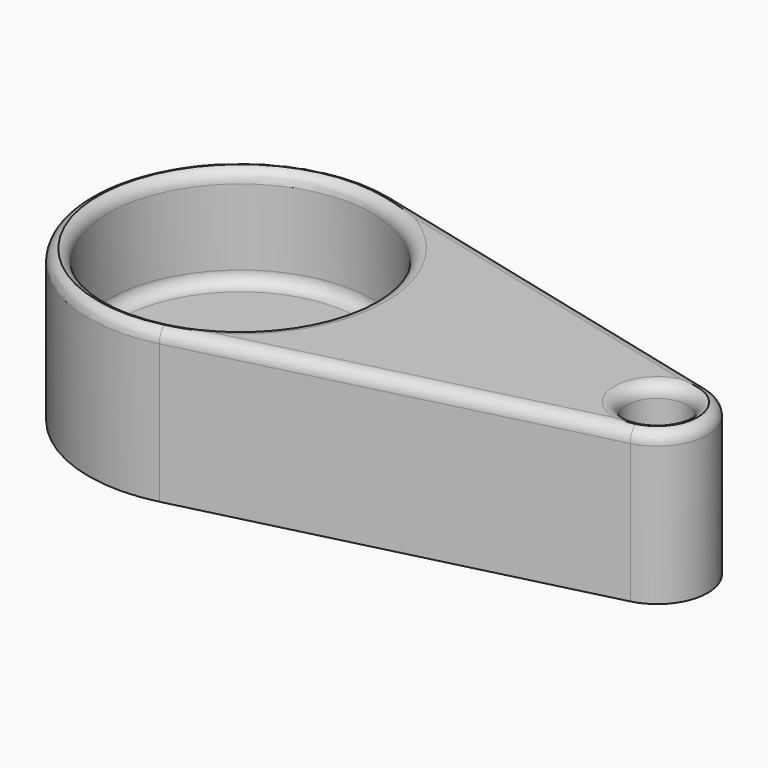
from build123d import *

# Parameters (mm, degrees)
F1_DEPTH     = 30
F2_R         = 26.25
F2_R_2       = 6
F3_DEPTH     = 20
F4_T5_DEPTH  = 80
F4_T7_DEPTH  = 80
F4_T10_ANGLE = 208.0724869359
F4_T12_ANGLE = 151.9275130641
F5_T         = -1


# Not quite as in the source:
# - a fillet or chamfer that OpenCascade refuses, or shapes differently, is made with other operations: its cross-section is extruded or revolved along the edge and cut away or added


with BuildPart() as f1:
    # F0 (on Top) → F1 (new body)
    with BuildSketch(Plane.XY):
        with BuildLine():
            ThreePointArc((-78.9887374496, -29.1042750044), (-62.6186430602, -18.4623662821), (-56.2648062007, 0))
            ThreePointArc((-56.2648062007, 0), (-62.6186430602, 18.4623662821), (-78.9887374496, 29.1042750044))
            ThreePointArc((-78.9887374496, 29.1042750044), (-116.2648062007, 0), (-78.9887374496, -29.1042750044))
        make_face()
        with BuildLine():
            ThreePointArc((-78.9887374496, 29.1042750044), (-62.6186430602, 18.4623662821), (-56.2648062007, 0))
            ThreePointArc((-56.2648062007, 0), (-62.6186430602, -18.4623662821), (-78.9887374496, -29.1042750044))
            Line((-78.9887374496, -29.1042750044), (-1.377337438, -9.7014250015))
            ThreePointArc((-1.377337438, -9.7014250015), (-13.8026936884, 0), (-1.377337438, 9.7014250015))
            Line((-1.377337438, 9.7014250015), (-78.9887374496, 29.1042750044))
        make_face()
        with BuildLine():
            ThreePointArc((6.1973063116, 0), (4.0793606918, 6.154122094), (-1.377337438, 9.7014250015))
            ThreePointArc((-1.377337438, 9.7014250015), (-13.8026936884, 0), (-1.377337438, -9.7014250015))
            ThreePointArc((-1.377337438, -9.7014250015), (4.0793606918, -6.154122094), (6.1973063116, 0))
        make_face()
    extrude(amount=F1_DEPTH)

    # F2 (on face) → F3 (cut)
    with BuildSketch(Plane.XY.offset(30)):
        with Locations((-86.2648062007, 0)):
            Circle(F2_R)
        with Locations((-3.8026936884, 0)):
            Circle(F2_R_2)
    extrude(amount=-F3_DEPTH, mode=Mode.SUBTRACT)

    # F4: fillet of radius 2.5 on 8 edges, made by hand

    # F4_s1 → F4_t2 (revolve)
    with BuildSketch(Plane.XZ):
        with BuildLine():
            ThreePointArc((-60.0148062007, 12.5), (-60.7470392478, 10.732233047), (-62.5148062007, 10))
            Line((-62.5148062007, 10), (-60.0148062007, 10))
            Line((-60.0148062007, 10), (-60.0148062007, 12.5))
        make_face()
    revolve(axis=Axis((-86.2648062007, 0, 10), (0, 0, 1)))

    # F4_s3 → F4_t4 (revolve)
    with BuildSketch(Plane.XZ):
        with BuildLine():
            ThreePointArc((2.1973063116, 12.5), (1.4650732646, 10.732233047), (-0.3026936884, 10))
            Line((-0.3026936884, 10), (2.1973063116, 10))
            Line((2.1973063116, 10), (2.1973063116, 12.5))
        make_face()
    revolve(axis=Axis((-3.8026936884, 0, 10), (0, 0, 1)))

    # F4_s6 → F4_t5 (cut)
    with BuildSketch(Plane(origin=(-3.5790058244, 0.8947514561, 0), x_dir=(0, 0, 1), z_dir=(-0.9701425001, 0.242535625, 0))):
        with BuildLine():
            ThreePointArc((27.5, 9.0777113095), (29.267766953, 8.3454782624), (30, 6.5777113095))
            Line((30, 6.5777113095), (30, 9.0777113095))
            Line((30, 9.0777113095), (27.5, 9.0777113095))
        make_face()
    extrude(amount=F4_T5_DEPTH, mode=Mode.SUBTRACT)

    # F4_s8 → F4_t7 (cut)
    with BuildSketch(Plane(origin=(-81.190405836, -20.297601459, 0), x_dir=(0, 0, 1), z_dir=(0.9701425001, 0.242535625, 0))):
        with BuildLine():
            ThreePointArc((27.5, 9.0777113095), (29.267766953, 8.3454782624), (30, 6.5777113095))
            Line((30, 6.5777113095), (30, 9.0777113095))
            Line((30, 9.0777113095), (27.5, 9.0777113095))
        make_face()
    extrude(amount=F4_T7_DEPTH, mode=Mode.SUBTRACT)

    # F4_s9 → F4_t10 (revolve, cut)
    with BuildSketch(Plane(origin=(-81.190405836, 20.297601459, 0), x_dir=(0, 0, 1), z_dir=(0.9701425001, -0.242535625, 0))):
        with BuildLine():
            ThreePointArc((27.5, -9.0777113095), (29.267766953, -8.3454782624), (30, -6.5777113095))
            Line((30, -6.5777113095), (30, -9.0777113095))
            Line((30, -9.0777113095), (27.5, -9.0777113095))
        make_face()
    revolve(axis=Axis((-86.2648062007, 0, 30), (0, 0, 1)), revolution_arc=F4_T10_ANGLE, mode=Mode.SUBTRACT)

    # F4_s11 → F4_t12 (revolve, cut)
    with BuildSketch(Plane(origin=(-3.5790058244, -0.8947514561, 0), x_dir=(0, 0, 1), z_dir=(-0.9701425001, -0.242535625, 0))):
        with BuildLine():
            ThreePointArc((30, -6.5777113095), (29.267766953, -8.3454782624), (27.5, -9.0777113095))
            Line((27.5, -9.0777113095), (30, -9.0777113095))
            Line((30, -9.0777113095), (30, -6.5777113095))
        make_face()
    revolve(axis=Axis((-3.8026936884, 0, 30), (0, 0, 1)), revolution_arc=F4_T12_ANGLE, mode=Mode.SUBTRACT)

    # F4_s13 → F4_t14 (revolve, cut)
    with BuildSketch(Plane.XZ):
        with BuildLine():
            ThreePointArc((-57.5148062007, 30), (-59.2825731537, 29.267766953), (-60.0148062007, 27.5))
            Line((-60.0148062007, 27.5), (-60.0148062007, 30))
            Line((-60.0148062007, 30), (-57.5148062007, 30))
        make_face()
    revolve(axis=Axis((-86.2648062007, 0, 30), (0, 0, 1)), mode=Mode.SUBTRACT)

    # F4_s15 → F4_t16 (revolve, cut)
    with BuildSketch(Plane.XZ):
        with BuildLine():
            ThreePointArc((4.6973063116, 30), (2.9295393587, 29.267766953), (2.1973063116, 27.5))
            Line((2.1973063116, 27.5), (2.1973063116, 30))
            Line((2.1973063116, 30), (4.6973063116, 30))
        make_face()
    revolve(axis=Axis((-3.8026936884, 0, 30), (0, 0, 1)), mode=Mode.SUBTRACT)

    # F5
    f5_openings = [f1.faces().sort_by_distance(p)[0] for p in [
        (-63.619436, 0, 0),
    ]]
    offset(amount=F5_T, openings=f5_openings)


solid = f1.part
